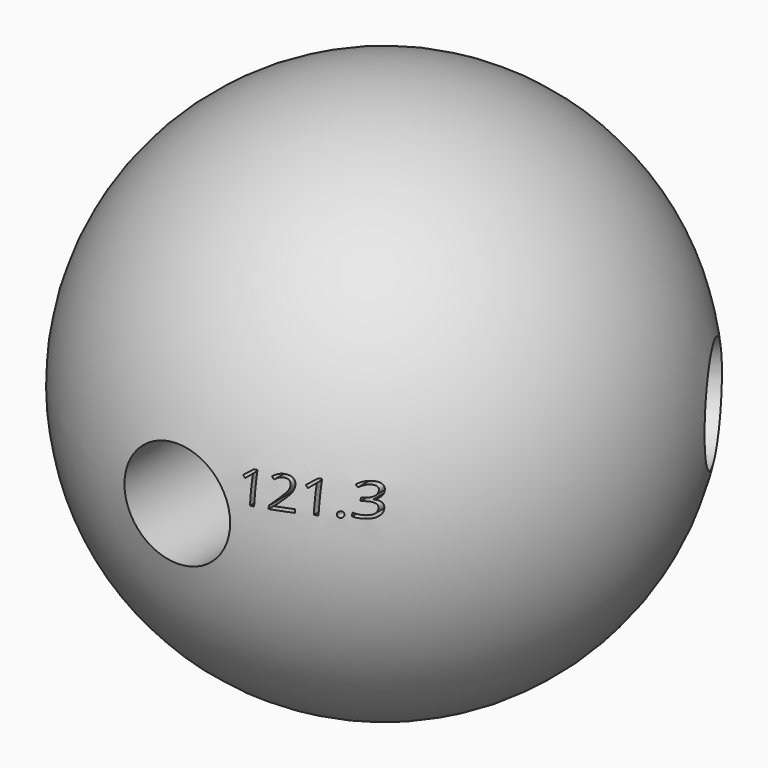
from build123d import *

# Parameters (mm, degrees)
F4_R          = 3.175
F5_DEPTH      = 25.4
F6_ANGLE      = -119.3
F7_ANGLE      = -119.4
F9_TEXT_SIZE  = 2.8734032336
F10_DEPTH     = 9.1186
F12_TEXT_SIZE = 2.6990548779
F13_DEPTH     = 8.0518
F16_TEXT_SIZE = 2.5663012315
F17_DEPTH     = 8.5344


# Not quite as in the source:
# - Text() gives the source's letters only with a copy of the font that has no kerning and outlines rounded to 1/6400 em; it was checked with that copy


with BuildPart() as f1:
    # F0 (on Top) → F1 (revolve)
    with BuildSketch(Plane.XY):
        with BuildLine():
            Line((0, -15.875), (0, 15.875))
            ThreePointArc((0, 15.875), (-15.875, 0), (0, -15.875))
        make_face()
    revolve(axis=Axis((0, 0, 0), (0, -1, 0)))

    # F9 (on offset) → F10 (cut)
    with BuildSketch(Plane(origin=(16.277440714, 9.8968390813, 0), x_dir=(-0.5195191119, 0.8544588301, 0), z_dir=(0.8544588301, 0.5195191119, 0))):
        with Locations((3.8055421319, 1.1255916907)):
            Text('119.4', F9_TEXT_SIZE, font='Open Sans', text_align=(TextAlign.LEFT, TextAlign.BOTTOM))
    extrude(amount=-F10_DEPTH, mode=Mode.SUBTRACT)

    # F12 (on offset) → F13 (cut)
    with BuildSketch(Plane(origin=(-16.6129196398, 9.3227357058, 0), x_dir=(-0.4893824517, -0.8720692724, 0), z_dir=(-0.8720692724, 0.4893824517, 0))):
        with Locations((3.7473766133, -0.5160869914)):
            Text('119.3', F12_TEXT_SIZE, font='Open Sans', text_align=(TextAlign.LEFT, TextAlign.BOTTOM))
    extrude(amount=-F13_DEPTH, mode=Mode.SUBTRACT)


with BuildPart() as f5:
    # F4 (on offset) → F5 (new body)
    with BuildSketch(Plane.XZ.offset(6.35)):
        Circle(F4_R)
    extrude(amount=F5_DEPTH)


with BuildPart() as f6_1:
    # F6: copy of F5
    add(f5.part.rotate(Axis((0, 0, 37.6308187842), (0, 0, 1)), F6_ANGLE))


with BuildPart() as f7_1:
    # F7: copy of F6_1
    add(f6_1.part.rotate(Axis((0, 0, 37.6308187842), (0, 0, 1)), F7_ANGLE))


with BuildPart() as f1_1:
    add(f1.part)

    # F14: cut F6_1, F5, F7_1
    add(f6_1.part, mode=Mode.SUBTRACT)
    add(f5.part, mode=Mode.SUBTRACT)
    add(f7_1.part, mode=Mode.SUBTRACT)

    # F16 (on offset) → F17 (cut)
    with BuildSketch(Plane.XZ.offset(19.685)):
        with Locations((3.4571681172, 1.1283926433)):
            Text('121.3', F16_TEXT_SIZE, font='Open Sans', text_align=(TextAlign.LEFT, TextAlign.BOTTOM))
    extrude(amount=-F17_DEPTH, mode=Mode.SUBTRACT)


solid = f1_1.part
